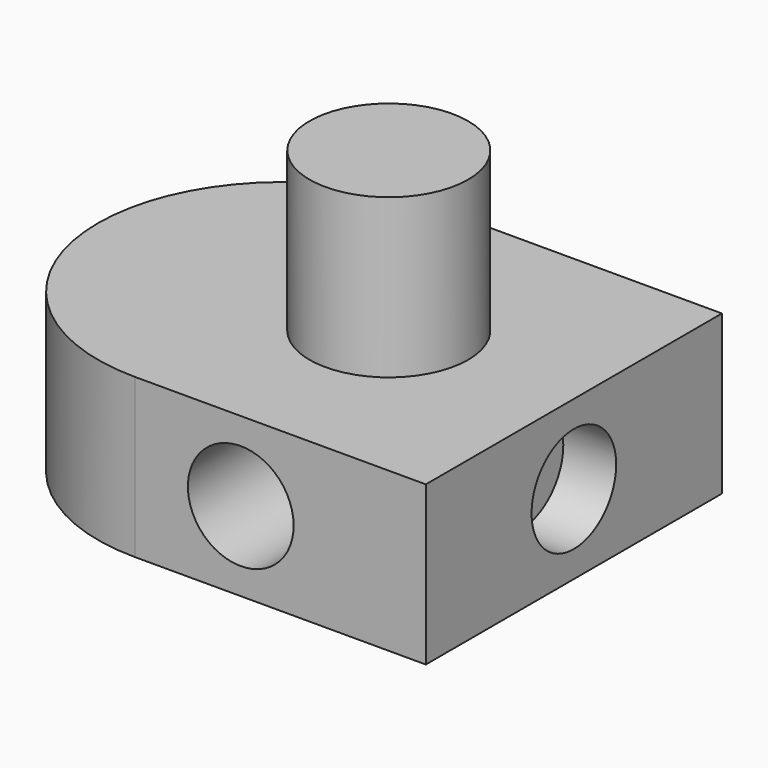
from build123d import *

# Parameters (mm, degrees)
F0_W           = 90
F0_H           = 70
F1_DEPTH       = 30
F2_R           = 34.99999
F3_R           = 10
F4_DEPTH       = 70.001
F6_D           = 10
F6_DEPTH       = 35
F6_CBORE_D     = 20
F6_CBORE_DEPTH = 10
F6_TIP         = 3.0043030951
F7_R           = 15
F8_DEPTH       = 30


# Not quite as in the source:
# - a fillet or chamfer is up to 0.001 mm smaller than in the source, because OpenCascade refuses the exact size


with BuildPart() as f1:
    # F0 (on Top) → F1 (new body)
    with BuildSketch(Plane.XY):
        Rectangle(F0_W, F0_H)
    extrude(amount=F1_DEPTH)

    # F2 (radius 35 in the source; OpenCascade refuses exactly that, so slightly less here)
    f2_edges = [f1.edges().sort_by_distance(p)[0] for p in [
        (-45, 35, 15),
        (-45, -35, 15),
    ]]
    fillet(f2_edges, radius=F2_R)

    # F3 (on face) → F4 (cut, through all)
    with BuildSketch(Plane.XZ.offset(35)):
        with Locations((10, 15)):
            Circle(F3_R)
    extrude(amount=-F4_DEPTH, mode=Mode.SUBTRACT)

    # F6
    with Locations(Plane.YZ.offset(45)):
        with Locations((0, 15)):
            CounterBoreHole(F6_D / 2, F6_CBORE_D / 2, F6_CBORE_DEPTH, depth=F6_DEPTH)
            with Locations((0, 0, -(F6_DEPTH + F6_TIP / 2))):  # 118° drill point
                Cone(0, F6_D / 2, F6_TIP, mode=Mode.SUBTRACT)

    # F7 (on face) → F8 (join)
    with BuildSketch(Plane.XY.offset(30)):
        with Locations((10, 0)):
            Circle(F7_R)
    extrude(amount=F8_DEPTH)


solid = f1.part
